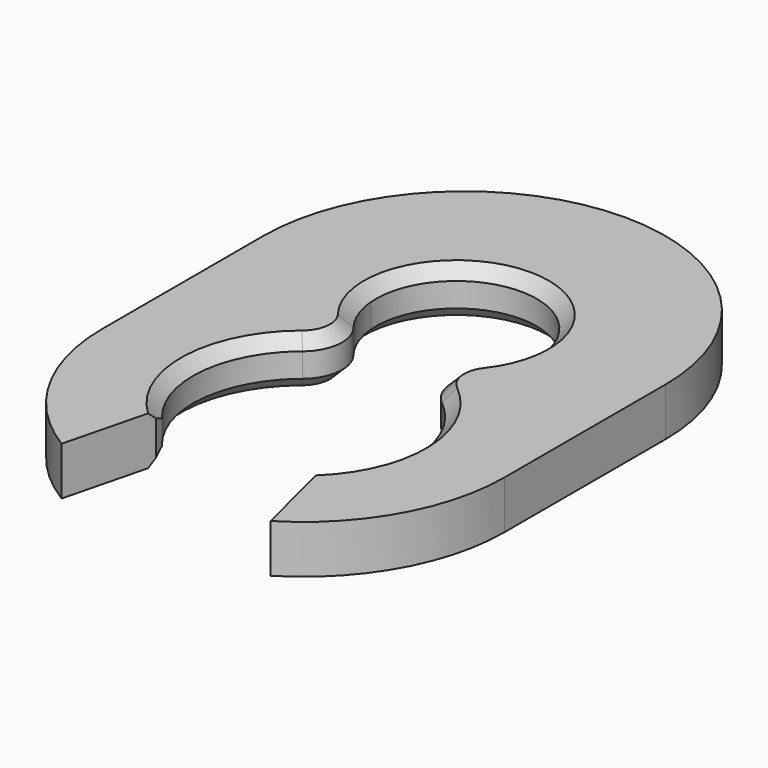
from build123d import *

# Parameters (mm, degrees)
F1_DEPTH     = 1.2
F2_T1_DEPTH  = 2.0490052379
F2_T4_ANGLE  = 110.2678169565
F2_T6_ANGLE  = 110.2678169565
F2_T8_ANGLE  = 110.2678169565
F2_T10_ANGLE = 110.2678169565
F2_T12_ANGLE = 255.7636829162
F2_T14_ANGLE = 255.7636829162
F2_T16_ANGLE = 88.7266556386
F2_T18_ANGLE = 88.7266556386
F2_T20_ANGLE = 88.7266556386
F2_T22_ANGLE = 88.7266556386


# Not quite as in the source:
# - a fillet or chamfer that OpenCascade refuses, or shapes differently, is made with other operations: its cross-section is extruded or revolved along the edge and cut away or added


with BuildPart() as f1:
    # F0 (on Top) → F1 (new body)
    with BuildSketch(Plane.XY):
        with BuildLine():
            Line((-2.6, -4.2708313008), (-2, -1.8874586088))
            ThreePointArc((-2, -1.8874586088), (-2.7441072414, 0.1799317859), (-1.7364132024, 2.1324561404))
            ThreePointArc((-1.7364132024, 2.1324561404), (-1.3742278026, 2.7950125758), (-1.5785574567, 3.5219298246))
            ThreePointArc((-1.5785574567, 3.5219298246), (-1.863388842, 4.0235139207), (-1.9932256288, 4.5855263158))
            ThreePointArc((-1.9932256288, 4.5855263158), (-4.1812754121, 2.7417031072), (-5, 0))
            ThreePointArc((-5, 0), (-4.3588989435, -2.4494897428), (-2.6, -4.2708313008))
        make_face()
        with BuildLine():
            ThreePointArc((1.7364132024, 2.1324561404), (2.4837105615, 1.1805430304), (2.75, 0))
            ThreePointArc((2.75, 0), (2.5556310375, -1.0155048006), (2, -1.8874586088))
            Line((2, -1.8874586088), (2.6, -4.2708313008))
            ThreePointArc((2.6, -4.2708313008), (4.3588989435, -2.4494897428), (5, 0))
            ThreePointArc((5, 0), (4.1812754121, 2.7417031072), (1.9932256288, 4.5855263158))
            ThreePointArc((1.9932256288, 4.5855263158), (1.863388842, 4.0235139207), (1.5785574567, 3.5219298246))
            ThreePointArc((1.5785574567, 3.5219298246), (1.3742278026, 2.7950125758), (1.7364132024, 2.1324561404))
        make_face()
        with BuildLine():
            ThreePointArc((2, 4.75), (1.9983056895, 4.6676934315), (1.9932256288, 4.5855263158))
            ThreePointArc((1.9932256288, 4.5855263158), (4.1812754121, 2.7417031072), (5, 0))
            Line((5, 0), (5, 5))
            ThreePointArc((5, 5), (0, 10), (-5, 5))
            Line((-5, 5), (-5, 0))
            ThreePointArc((-5, 0), (-4.1812754121, 2.7417031072), (-1.9932256288, 4.5855263158))
            ThreePointArc((-1.9932256288, 4.5855263158), (-0.0823065685, 6.7483056895), (2, 4.75))
        make_face()
    extrude(amount=F1_DEPTH)

    # F2: chamfer of 0.3 on 12 edges, made by hand

    # F2_s2 → F2_t1 (cut)
    with BuildSketch(Plane.XY.offset(-0.4245026189)):
        with BuildLine():
            Line((-2.0361189998, -2.0533736883), (-2.103298477, -1.7631362182))
            Line((-2.103298477, -1.7631362182), (-2.0987153662, -1.7592638681))
            ThreePointArc((-2.0987153662, -1.7592638681), (-2.0500925283, -1.8239124501), (-1.9956363636, -1.8833405173))
            Line((-1.9956363636, -1.8833405173), (-1.9941815406, -1.8889233716))
            ThreePointArc((-1.9941815406, -1.8889233716), (-2.0148972724, -1.9712122207), (-2.0303005404, -2.0548384511))
            Line((-2.0303005404, -2.0548384511), (-2.0361189998, -2.0533736883))
        make_face()
        with BuildLine():
            Line((2.103298477, -1.7631362182), (2.0361189998, -2.0533736883))
            Line((2.0361189998, -2.0533736883), (2.0303005404, -2.0548384511))
            ThreePointArc((2.0303005404, -2.0548384511), (2.0148972724, -1.9712122207), (1.9941815406, -1.8889233716))
            Line((1.9941815406, -1.8889233716), (1.9956363636, -1.8833405173))
            ThreePointArc((1.9956363636, -1.8833405173), (2.0500925283, -1.8239124501), (2.0987153662, -1.7592638681))
            Line((2.0987153662, -1.7592638681), (2.103298477, -1.7631362182))
        make_face()
    extrude(amount=F2_T1_DEPTH, mode=Mode.SUBTRACT)

    # F2_s3 → F2_t4 (revolve, cut)
    with BuildSketch(Plane(origin=(0, 0, 0), x_dir=(0, 0, 1), z_dir=(0.8609463246, -0.508695809, 0))):
        with BuildLine():
            Line((0.8915147186, 2.7415147186), (1.2084852814, 3.0584852814))
            Line((1.2084852814, 3.0584852814), (1.2144852814, 3.0584852814))
            ThreePointArc((1.2144852814, 3.0584852814), (1.206, 2.9042426407), (1.206, 2.75))
            Line((1.206, 2.75), (1.2, 2.744))
            ThreePointArc((1.2, 2.744), (1.0457573593, 2.744), (0.8915147186, 2.7355147186))
            Line((0.8915147186, 2.7355147186), (0.8915147186, 2.7415147186))
        make_face()
    revolve(axis=Axis((0, 0, 1.2), (0, 0, -1)), revolution_arc=F2_T4_ANGLE, mode=Mode.SUBTRACT)

    # F2_s5 → F2_t6 (revolve, cut)
    with BuildSketch(Plane(origin=(0, 0, 0), x_dir=(0, 0, 1), z_dir=(0.8609463246, -0.508695809, 0))):
        with BuildLine():
            Line((0.3084852814, 2.7415147186), (-0.0084852814, 3.0584852814))
            Line((-0.0084852814, 3.0584852814), (-0.0144852814, 3.0584852814))
            ThreePointArc((-0.0144852814, 3.0584852814), (-0.006, 2.9042426407), (-0.006, 2.75))
            Line((-0.006, 2.75), (0, 2.744))
            ThreePointArc((0, 2.744), (0.1542426407, 2.744), (0.3084852814, 2.7355147186))
            Line((0.3084852814, 2.7355147186), (0.3084852814, 2.7415147186))
        make_face()
    revolve(axis=Axis((0, 0, 0), (0, 0, -1)), revolution_arc=F2_T6_ANGLE, mode=Mode.SUBTRACT)

    # F2_s7 → F2_t8 (revolve, cut)
    with BuildSketch(Plane(origin=(0, 0, 0), x_dir=(0, 0, 1), z_dir=(-0.7754385965, 0.6314229827, 0))):
        with BuildLine():
            Line((0.8915147186, 2.7415147186), (1.2084852814, 3.0584852814))
            Line((1.2084852814, 3.0584852814), (1.2144852814, 3.0584852814))
            ThreePointArc((1.2144852814, 3.0584852814), (1.206, 2.9042426407), (1.206, 2.75))
            Line((1.206, 2.75), (1.2, 2.744))
            ThreePointArc((1.2, 2.744), (1.0457573593, 2.744), (0.8915147186, 2.7355147186))
            Line((0.8915147186, 2.7355147186), (0.8915147186, 2.7415147186))
        make_face()
    revolve(axis=Axis((0, 0, 1.2), (0, 0, -1)), revolution_arc=F2_T8_ANGLE, mode=Mode.SUBTRACT)

    # F2_s9 → F2_t10 (revolve, cut)
    with BuildSketch(Plane(origin=(0, 0, 0), x_dir=(0, 0, 1), z_dir=(-0.7754385965, 0.6314229827, 0))):
        with BuildLine():
            Line((0.3084852814, 2.7415147186), (-0.0084852814, 3.0584852814))
            Line((-0.0084852814, 3.0584852814), (-0.0144852814, 3.0584852814))
            ThreePointArc((-0.0144852814, 3.0584852814), (-0.006, 2.9042426407), (-0.006, 2.75))
            Line((-0.006, 2.75), (0, 2.744))
            ThreePointArc((0, 2.744), (0.1542426407, 2.744), (0.3084852814, 2.7355147186))
            Line((0.3084852814, 2.7355147186), (0.3084852814, 2.7415147186))
        make_face()
    revolve(axis=Axis((0, 0, 0), (0, 0, -1)), revolution_arc=F2_T10_ANGLE, mode=Mode.SUBTRACT)

    # F2_s11 → F2_t12 (revolve, cut)
    with BuildSketch(Plane(origin=(-2.3020629577, 2.9590643275, 0), x_dir=(0, 0, 1), z_dir=(0.6140350877, -0.7892787284, 0))):
        with BuildLine():
            Line((0.8915147186, -0.925151948), (1.2084852814, -0.6081813853))
            Line((1.2084852814, -0.6081813853), (1.2144852814, -0.6081813853))
            ThreePointArc((1.2144852814, -0.6081813853), (1.206, -0.762424026), (1.206, -0.9166666667))
            Line((1.206, -0.9166666667), (1.2, -0.9226666667))
            ThreePointArc((1.2, -0.9226666667), (1.0457573593, -0.9226666667), (0.8915147186, -0.931151948))
            Line((0.8915147186, -0.931151948), (0.8915147186, -0.925151948))
        make_face()
    revolve(axis=Axis((0, 4.75, 1.2), (0, 0, -1)), revolution_arc=F2_T12_ANGLE, mode=Mode.SUBTRACT)

    # F2_s13 → F2_t14 (revolve, cut)
    with BuildSketch(Plane(origin=(-2.3020629577, 2.9590643275, 0), x_dir=(0, 0, 1), z_dir=(0.6140350877, -0.7892787284, 0))):
        with BuildLine():
            Line((0.3084852814, -0.925151948), (-0.0084852814, -0.6081813853))
            Line((-0.0084852814, -0.6081813853), (-0.0144852814, -0.6081813853))
            ThreePointArc((-0.0144852814, -0.6081813853), (-0.006, -0.762424026), (-0.006, -0.9166666667))
            Line((-0.006, -0.9166666667), (0, -0.9226666667))
            ThreePointArc((0, -0.9226666667), (0.1542426407, -0.9226666667), (0.3084852814, -0.931151948))
            Line((0.3084852814, -0.931151948), (0.3084852814, -0.925151948))
        make_face()
    revolve(axis=Axis((0, 4.75, 0), (0, 0, -1)), revolution_arc=F2_T14_ANGLE, mode=Mode.SUBTRACT)

    # F2_s15 → F2_t16 (revolve, cut)
    with BuildSketch(Plane(origin=(0, 0, 0), x_dir=(0, 0, 1), z_dir=(-0.7754385965, -0.6314229827, 0))):
        with BuildLine():
            Line((0.8915147186, 2.7415147186), (1.2084852814, 3.0584852814))
            Line((1.2084852814, 3.0584852814), (1.2144852814, 3.0584852814))
            ThreePointArc((1.2144852814, 3.0584852814), (1.206, 2.9042426407), (1.206, 2.75))
            Line((1.206, 2.75), (1.2, 2.744))
            ThreePointArc((1.2, 2.744), (1.0457573593, 2.744), (0.8915147186, 2.7355147186))
            Line((0.8915147186, 2.7355147186), (0.8915147186, 2.7415147186))
        make_face()
    revolve(axis=Axis((-2.3678361851, 2.9078947368, 1.2), (0, 0, 1)), revolution_arc=F2_T16_ANGLE, mode=Mode.SUBTRACT)

    # F2_s17 → F2_t18 (revolve, cut)
    with BuildSketch(Plane(origin=(0, 0, 0), x_dir=(0, 0, 1), z_dir=(-0.7754385965, -0.6314229827, 0))):
        with BuildLine():
            Line((0.3084852814, 2.7415147186), (-0.0084852814, 3.0584852814))
            Line((-0.0084852814, 3.0584852814), (-0.0144852814, 3.0584852814))
            ThreePointArc((-0.0144852814, 3.0584852814), (-0.006, 2.9042426407), (-0.006, 2.75))
            Line((-0.006, 2.75), (0, 2.744))
            ThreePointArc((0, 2.744), (0.1542426407, 2.744), (0.3084852814, 2.7355147186))
            Line((0.3084852814, 2.7355147186), (0.3084852814, 2.7415147186))
        make_face()
    revolve(axis=Axis((-2.3678361851, 2.9078947368, 0), (0, 0, 1)), revolution_arc=F2_T18_ANGLE, mode=Mode.SUBTRACT)

    # F2_s19 → F2_t20 (revolve, cut)
    with BuildSketch(Plane(origin=(2.3020629577, 2.9590643275, 0), x_dir=(0, 0, 1), z_dir=(0.6140350877, 0.7892787284, 0))):
        with BuildLine():
            Line((0.8915147186, -0.925151948), (1.2084852814, -0.6081813853))
            Line((1.2084852814, -0.6081813853), (1.2144852814, -0.6081813853))
            ThreePointArc((1.2144852814, -0.6081813853), (1.206, -0.762424026), (1.206, -0.9166666667))
            Line((1.206, -0.9166666667), (1.2, -0.9226666667))
            ThreePointArc((1.2, -0.9226666667), (1.0457573593, -0.9226666667), (0.8915147186, -0.931151948))
            Line((0.8915147186, -0.931151948), (0.8915147186, -0.925151948))
        make_face()
    revolve(axis=Axis((2.3678361851, 2.9078947368, 1.2), (0, 0, 1)), revolution_arc=F2_T20_ANGLE, mode=Mode.SUBTRACT)

    # F2_s21 → F2_t22 (revolve, cut)
    with BuildSketch(Plane(origin=(2.3020629577, 2.9590643275, 0), x_dir=(0, 0, 1), z_dir=(0.6140350877, 0.7892787284, 0))):
        with BuildLine():
            Line((0.3084852814, -0.925151948), (-0.0084852814, -0.6081813853))
            Line((-0.0084852814, -0.6081813853), (-0.0144852814, -0.6081813853))
            ThreePointArc((-0.0144852814, -0.6081813853), (-0.006, -0.762424026), (-0.006, -0.9166666667))
            Line((-0.006, -0.9166666667), (0, -0.9226666667))
            ThreePointArc((0, -0.9226666667), (0.1542426407, -0.9226666667), (0.3084852814, -0.931151948))
            Line((0.3084852814, -0.931151948), (0.3084852814, -0.925151948))
        make_face()
    revolve(axis=Axis((2.3678361851, 2.9078947368, 0), (0, 0, 1)), revolution_arc=F2_T22_ANGLE, mode=Mode.SUBTRACT)


solid = f1.part
